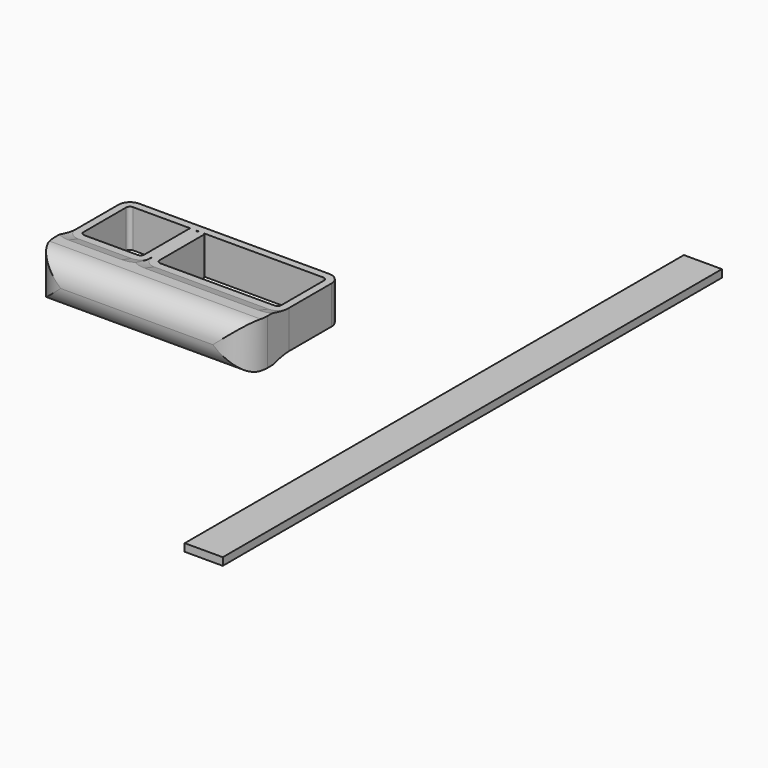
from build123d import *

# Parameters (mm, degrees)
F1_DEPTH      = 15.875
F3_DEPTH      = 17.4625
F3_DEPTH_BACK = 1.5875
F4_T1_DEPTH   = 22.225
F4_T3_DEPTH   = 47.625
F4_T6_ANGLE   = 248.6962956801
F4_T8_ANGLE   = 248.6962956801
F4_T10_ANGLE  = 248.6962956801
F4_T12_ANGLE  = 248.6962956801
F4_T14_ANGLE  = 248.6962956801
F4_T16_ANGLE  = 248.6962956801
F4_T18_ANGLE  = 248.6962956801
F4_T20_ANGLE  = 248.6962956801
F6_T1_DEPTH   = 111.125
F7_W          = 15.875
F7_H          = 25.4
F7_H_2        = 82.55
F7_H_3        = 50.8
F8_DEPTH      = 3.175


# Not quite as in the source:
# - a fillet or chamfer that OpenCascade refuses, or shapes differently, is made with other operations: its cross-section is extruded or revolved along the edge and cut away or added
# - two fillets or chamfers of one size are made in one step
# - the program builds the solid bodies; features that only make, move or delete a surface that nothing else refers to are left out


with BuildPart() as f1:
    # F0 (on Top) → F1 (new body)
    with BuildSketch(Plane.XY):
        with BuildLine():
            ThreePointArc((-4.7625, -3.175), (-1.3949039546, -1.7800960454), (0, 1.5875))
            ThreePointArc((0, 1.5875), (1.3949039546, -1.7800960454), (4.7625, -3.175))
            Line((4.7625, -3.175), (52.3875, -3.175))
            ThreePointArc((52.3875, -3.175), (55.7550960454, -1.7800960454), (57.15, 1.5875))
            Line((57.15, 1.5875), (57.15, 23.8125))
            ThreePointArc((57.15, 23.8125), (55.7550960454, 27.1800960454), (52.3875, 28.575))
            Line((52.3875, 28.575), (-26.9875, 28.575))
            ThreePointArc((-26.9875, 28.575), (-30.3550960454, 27.1800960454), (-31.75, 23.8125))
            Line((-31.75, 23.8125), (-31.75, 1.5875))
            ThreePointArc((-31.75, 1.5875), (-30.3550960454, -1.7800960454), (-26.9875, -3.175))
            Line((-26.9875, -3.175), (-4.7625, -3.175))
        make_face()
        with BuildLine():
            Line((-4.7625, 0), (-26.9875, 0))
            ThreePointArc((-26.9875, 0), (-28.1100320151, 0.4649679849), (-28.575, 1.5875))
            Line((-28.575, 1.5875), (-28.575, 23.8125))
            ThreePointArc((-28.575, 23.8125), (-28.1100320151, 24.9350320151), (-26.9875, 25.4))
            Line((-26.9875, 25.4), (-2.37998, 25.4))
            ThreePointArc((-2.37998, 25.4), (-2.9421440332, 25.1671440332), (-3.175, 24.60498))
            Line((-3.175, 24.60498), (-3.175, 1.5875))
            ThreePointArc((-3.175, 1.5875), (-3.6399679849, 0.4649679849), (-4.7625, 0))
        make_face(mode=Mode.SUBTRACT)
        with BuildLine():
            ThreePointArc((0, 24.60498), (-0.2328559668, 25.1671440332), (-0.79502, 25.4))
            Line((-0.79502, 25.4), (0.79502, 25.4))
            ThreePointArc((0.79502, 25.4), (0.2328559668, 25.1671440332), (0, 24.60498))
        make_face(mode=Mode.SUBTRACT)
        with BuildLine():
            ThreePointArc((3.175, 24.60498), (2.9421440332, 25.1671440332), (2.37998, 25.4))
            Line((2.37998, 25.4), (52.3875, 25.4))
            ThreePointArc((52.3875, 25.4), (53.5100320151, 24.9350320151), (53.975, 23.8125))
            Line((53.975, 23.8125), (53.975, 1.5875))
            ThreePointArc((53.975, 1.5875), (53.5100320151, 0.4649679849), (52.3875, 0))
            Line((52.3875, 0), (4.7625, 0))
            ThreePointArc((4.7625, 0), (3.6399679849, 0.4649679849), (3.175, 1.5875))
            Line((3.175, 1.5875), (3.175, 24.60498))
        make_face(mode=Mode.SUBTRACT)
    extrude(amount=F1_DEPTH)


with BuildPart() as f3:
    # F0 (on Top) → F3 (new body, two sides)
    with BuildSketch(Plane.XY) as f3_sk:
        with BuildLine():
            Line((52.3875, -3.175), (4.7625, -3.175))
            Line((4.7625, -3.175), (-4.7625, -3.175))
            Line((-4.7625, -3.175), (-26.9875, -3.175))
            Line((-26.9875, -3.175), (-31.75, -3.175))
            Line((-31.75, -3.175), (-31.75, -9.525))
            ThreePointArc((-31.75, -9.525), (-28.0302561211, -18.5052561211), (-19.05, -22.225))
            Line((-19.05, -22.225), (44.45, -22.225))
            ThreePointArc((44.45, -22.225), (53.4302561211, -18.5052561211), (57.15, -9.525))
            Line((57.15, -9.525), (57.15, -3.175))
            Line((57.15, -3.175), (52.3875, -3.175))
        make_face()
        with BuildLine():
            ThreePointArc((4.7625, -3.175), (1.3949039546, -1.7800960454), (0, 1.5875))
            ThreePointArc((0, 1.5875), (-1.3949039546, -1.7800960454), (-4.7625, -3.175))
            Line((-4.7625, -3.175), (4.7625, -3.175))
        make_face()
        with BuildLine():
            ThreePointArc((57.15, 1.5875), (55.7550960454, -1.7800960454), (52.3875, -3.175))
            Line((52.3875, -3.175), (57.15, -3.175))
            Line((57.15, -3.175), (57.15, 1.5875))
        make_face()
        with BuildLine():
            Line((-31.75, -3.175), (-26.9875, -3.175))
            ThreePointArc((-26.9875, -3.175), (-30.3550960454, -1.7800960454), (-31.75, 1.5875))
            Line((-31.75, 1.5875), (-31.75, -3.175))
        make_face()
    extrude(amount=F3_DEPTH)
    extrude(f3_sk.sketch, amount=-F3_DEPTH_BACK)

    # F4: chamfer of 1.5875 x 5.08 on 8 edges, made by hand

    # F4_s2 → F4_t1 (cut)
    with BuildSketch(Plane.YZ.offset(-26.9875)):
        Polygon((-3.175, 15.875), (-8.255, 17.4625), (-3.175, 17.4625), align=None)
        Polygon((-8.255, -1.5875), (-3.175, 0), (-3.175, -1.5875), align=None)
    extrude(amount=F4_T1_DEPTH, mode=Mode.SUBTRACT)

    # F4_s4 → F4_t3 (cut)
    with BuildSketch(Plane.YZ.offset(4.7625)):
        Polygon((-3.175, 15.875), (-8.255, 17.4625), (-3.175, 17.4625), align=None)
        Polygon((-8.255, -1.5875), (-3.175, 0), (-3.175, -1.5875), align=None)
    extrude(amount=F4_T3_DEPTH, mode=Mode.SUBTRACT)

    # F4_s5 → F4_t6 (revolve, cut)
    with BuildSketch(Plane.YZ.offset(-26.9875)):
        Polygon((-3.175, 15.875), (-8.255, 17.4625), (-3.175, 17.4625), align=None)
    revolve(axis=Axis((-26.9875, 1.5875, 17.4625), (0, 0, -1)), revolution_arc=F4_T6_ANGLE, mode=Mode.SUBTRACT)

    # F4_s7 → F4_t8 (revolve, cut)
    with BuildSketch(Plane.YZ.offset(4.7625)):
        Polygon((-3.175, 15.875), (-8.255, 17.4625), (-3.175, 17.4625), align=None)
    revolve(axis=Axis((4.7625, 1.5875, 17.4625), (0, 0, -1)), revolution_arc=F4_T8_ANGLE, mode=Mode.SUBTRACT)

    # F4_s9 → F4_t10 (revolve, cut)
    with BuildSketch(Plane(origin=(-0.0912813949, -0.2340799532, 0), x_dir=(0, 0, 1), z_dir=(-0.363311466, -0.9316677405, 0))):
        Polygon((15.875, 9.7763245664), (17.4625, 14.8563245664), (17.4625, 9.7763245664), align=None)
    revolve(axis=Axis((-4.7625, 1.5875, 17.4625), (0, 0, -1)), revolution_arc=F4_T10_ANGLE, mode=Mode.SUBTRACT)

    # F4_s11 → F4_t12 (revolve, cut)
    with BuildSketch(Plane(origin=(7.452245502, 19.1103705201, 0), x_dir=(0, 0, 1), z_dir=(-0.363311466, -0.9316677405, 0))):
        Polygon((15.875, -43.4684868037), (17.4625, -38.3884868037), (17.4625, -43.4684868037), align=None)
    revolve(axis=Axis((52.3875, 1.5875, 17.4625), (0, 0, -1)), revolution_arc=F4_T12_ANGLE, mode=Mode.SUBTRACT)

    # F4_s13 → F4_t14 (revolve, cut)
    with BuildSketch(Plane(origin=(-0.0912813949, -0.2340799532, 0), x_dir=(0, 0, 1), z_dir=(-0.363311466, -0.9316677405, 0))):
        Polygon((-1.5875, 14.8563245664), (0, 9.7763245664), (-1.5875, 9.7763245664), align=None)
    revolve(axis=Axis((-4.7625, 1.5875, -1.5875), (0, 0, -1)), revolution_arc=F4_T14_ANGLE, mode=Mode.SUBTRACT)

    # F4_s15 → F4_t16 (revolve, cut)
    with BuildSketch(Plane.YZ.offset(-26.9875)):
        Polygon((-8.255, -1.5875), (-3.175, 0), (-3.175, -1.5875), align=None)
    revolve(axis=Axis((-26.9875, 1.5875, -1.5875), (0, 0, -1)), revolution_arc=F4_T16_ANGLE, mode=Mode.SUBTRACT)

    # F4_s17 → F4_t18 (revolve, cut)
    with BuildSketch(Plane(origin=(7.452245502, 19.1103705201, 0), x_dir=(0, 0, 1), z_dir=(-0.363311466, -0.9316677405, 0))):
        Polygon((-1.5875, -38.3884868037), (0, -43.4684868037), (-1.5875, -43.4684868037), align=None)
    revolve(axis=Axis((52.3875, 1.5875, -1.5875), (0, 0, -1)), revolution_arc=F4_T18_ANGLE, mode=Mode.SUBTRACT)

    # F4_s19 → F4_t20 (revolve, cut)
    with BuildSketch(Plane.YZ.offset(4.7625)):
        Polygon((-8.255, -1.5875), (-3.175, 0), (-3.175, -1.5875), align=None)
    revolve(axis=Axis((4.7625, 1.5875, -1.5875), (0, 0, -1)), revolution_arc=F4_T20_ANGLE, mode=Mode.SUBTRACT)

    # F6: fillet of radius 9.525 on 4 edges, made by hand

    # F6_s2 → F6_t1 (cut)
    with BuildSketch(Plane.YZ.offset(-42.8625)):
        with BuildLine():
            ThreePointArc((-22.225, 7.9375), (-19.4351920908, 14.6726920908), (-12.7, 17.4625))
            Line((-12.7, 17.4625), (-22.225, 17.4625))
            Line((-22.225, 17.4625), (-22.225, 7.9375))
        make_face()
        with BuildLine():
            ThreePointArc((-22.225, 7.9375), (-19.4351920908, 1.2023079092), (-12.7, -1.5875))
            Line((-12.7, -1.5875), (-22.225, -1.5875))
            Line((-22.225, -1.5875), (-22.225, 7.9375))
        make_face()
    extrude(amount=F6_T1_DEPTH, mode=Mode.SUBTRACT)


with BuildPart() as f8:
    # F7 (on Top) → F8 (new body)
    with BuildSketch(Plane.XY):
        with Locations((127, -117.475)):
            Rectangle(F7_W, F7_H)
        with Locations((127, -92.075)):
            Rectangle(F7_W, F7_H)
        with Locations((127, -66.675)):
            Rectangle(F7_W, F7_H)
        with Locations((127, -12.7)):
            Rectangle(F7_W, F7_H_2)
        with Locations((127, 41.275)):
            Rectangle(F7_W, F7_H)
        with Locations((127, 79.375)):
            Rectangle(F7_W, F7_H_3)
        with Locations((127, 117.475)):
            Rectangle(F7_W, F7_H)
    extrude(amount=F8_DEPTH)


solid = Compound([f1.part, f3.part, f8.part])
